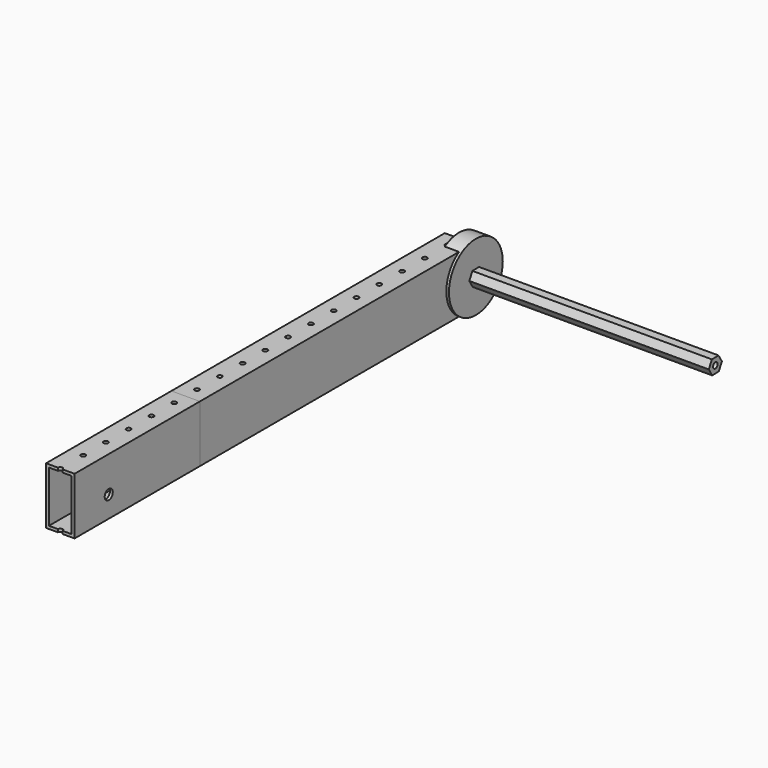
from build123d import *

# Parameters (mm, degrees)
F0_W      = 25.4
F0_H      = 50.8
F0_W_2    = 20.32
F0_H_2    = 45.72
F1_DEPTH  = 444.5
F4_D      = 9
F5_R      = 30
F6_DEPTH  = 15
F7_DEPTH  = 304.8
F2_R      = 2.0701
F8_DEPTH  = 55.401
F10_DEPTH = 228.6
F11_D     = 5.1054
F12_D     = 4.4958


with BuildPart() as f1:
    # F0 (on Front) → F1 (new body)
    with BuildSketch(Plane.XZ):
        Rectangle(F0_W, F0_H)
        Rectangle(F0_W_2, F0_H_2, mode=Mode.SUBTRACT)
    extrude(amount=F1_DEPTH)

    # F4 (through all)
    with Locations(Plane.YZ.offset(12.7)):
        with Locations((-406.4, -6.35), (-222.25, -7.9375), (-38.1, -6.35)):
            Hole(F4_D / 2)


with BuildPart() as f6:
    # F5 (on Right) → F6 (new body)
    with BuildSketch(Plane.YZ):
        Circle(F5_R)
    extrude(amount=F6_DEPTH)


with BuildPart() as f7:
    # F0 (on Front) → F7 (new body)
    with BuildSketch(Plane.XZ):
        Rectangle(F0_W, F0_H)
        Rectangle(F0_W_2, F0_H_2, mode=Mode.SUBTRACT)
    extrude(amount=F7_DEPTH)


with BuildPart() as f8_tool:
    # F2 (on face) → F8 (new body, through all)
    with BuildSketch(Plane.XY.offset(25.4)):
        with Locations((0, -12.7)):
            Circle(F2_R)
        with Locations((0, -38.1)):
            Circle(F2_R)
        with Locations((0, -63.5)):
            Circle(F2_R)
        with Locations((0, -88.9)):
            Circle(F2_R)
        with Locations((0, -114.3)):
            Circle(F2_R)
        with Locations((0, -139.7)):
            Circle(F2_R)
        with Locations((0, -165.1)):
            Circle(F2_R)
        with Locations((0, -190.5)):
            Circle(F2_R)
        with Locations((0, -215.9)):
            Circle(F2_R)
        with Locations((0, -241.3)):
            Circle(F2_R)
        with Locations((0, -266.7)):
            Circle(F2_R)
        with Locations((0, -292.1)):
            Circle(F2_R)
        with Locations((0, -317.5)):
            Circle(F2_R)
        with Locations((0, -342.9)):
            Circle(F2_R)
        with Locations((0, -368.3)):
            Circle(F2_R)
        with Locations((0, -393.7)):
            Circle(F2_R)
        with Locations((0, -419.1)):
            Circle(F2_R)
        with Locations((0, -444.5)):
            Circle(F2_R)
    extrude(amount=-F8_DEPTH)


with BuildPart() as f1_1:
    add(f1.part)

    # F8: cut by f8_tool
    add(f8_tool.part, mode=Mode.SUBTRACT)

    # F12 (through all)
    with Locations(Plane.YZ.offset(12.7)):
        with Locations((-260.35, 19.05), (-184.15, 19.05), (-184.15, -19.05), (-260.35, -19.05)):
            Hole(F12_D / 2)


with BuildPart() as f7_1:
    add(f7.part)

    # F8: cut by f8_tool
    add(f8_tool.part, mode=Mode.SUBTRACT)


with BuildPart() as f10:
    # F9 (on Right) → F10 (new body)
    with BuildSketch(Plane.YZ):
        Polygon((3.7952121831, -6.2737307735), (7.3308163179, 0.1498847766), (3.5356041348, 6.4236155501), (-3.7952121831, 6.2737307735), (-7.3308163179, -0.1498847766), (-3.5356041348, -6.4236155501), align=None)
    extrude(amount=F10_DEPTH)

    # F11 (through all)
    with Locations(Plane(origin=(0, 0, 0), x_dir=(0, 1, 0), z_dir=(-1, 0, 0))):
        with Locations((0, 0)):
            Hole(F11_D / 2)


solid = Compound([f6.part, f1_1.part, f7_1.part, f10.part])
